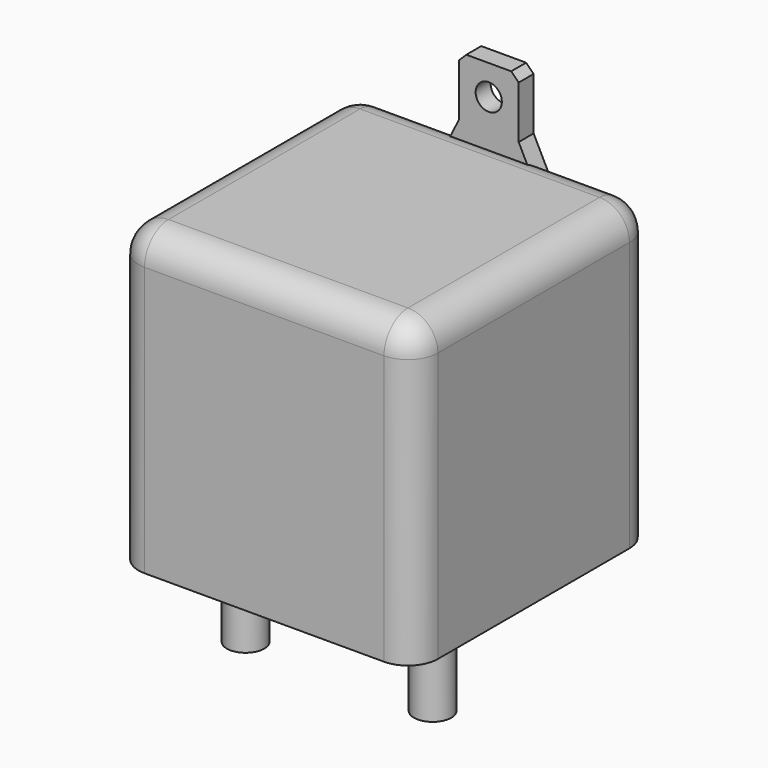
from build123d import *

# Parameters (mm, degrees)
F0_W         = 50.8
F0_H         = 50.8
F1_DEPTH     = 50.8
F2_R         = 2.2225
F3_DEPTH     = 3.175
F5_R         = 5.08
F6_T1_DEPTH  = 40.64
F6_T3_DEPTH  = 58.42
F6_T6_ANGLE  = 90
F6_T10_DEPTH = 26.67
F6_T16_DEPTH = 26.67
F6_T22_DEPTH = 26.67
F6_T27_ANGLE = 90
F6_T31_DEPTH = 26.67
F6_T38_DEPTH = 26.67
F6_T44_DEPTH = 26.67
F6_T48_ANGLE = 90
F6_T50_ANGLE = 90
F7_R         = 3.175
F8_DEPTH     = 15.24
F7_W         = 1.27
F7_H         = 6.35
F9_DEPTH     = 8.255


# Not quite as in the source:
# - a fillet or chamfer that OpenCascade refuses, or shapes differently, is made with other operations: its cross-section is extruded or revolved along the edge and cut away or added
# - a feature of the source that left no trace in its solid (it failed there, or was rolled back) is left out


with BuildPart() as f1:
    # F0 (on Top) → F1 (new body)
    with BuildSketch(Plane.XY):
        with Locations((-4.6946440548, -2.4632510453)):
            Rectangle(F0_W, F0_H)
    extrude(amount=F1_DEPTH)

    # F2 (on face) → F3 (join)
    with BuildSketch(Plane(origin=(0, 22.9367489547, 0), x_dir=(-1, 0, 0), z_dir=(0, 1, 0))):
        Polygon((-0.3853559452, 62.23), (-0.3853559452, 53.34), (9.7746440548, 53.34), (9.7746440548, 62.23), (8.5046440548, 63.5), (0.8846440548, 63.5), align=None)
        with Locations((4.6946440548, 58.42)):
            Circle(F2_R, mode=Mode.SUBTRACT)
        Polygon((-0.3853559452, 53.34), (-1.6553559452, 50.8), (11.0446440548, 50.8), (9.7746440548, 53.34), align=None)
    extrude(amount=-F3_DEPTH)

    # F5
    f5_edges = [f1.edges().sort_by_distance(p)[0] for p in [
        (-30.094644, -2.463251, 50.8),
        (20.705356, -2.463251, 50.8),
    ]]
    fillet(f5_edges, radius=F5_R)

    # F6: fillet of radius 5.08 on 11 edges, made by hand

    # F6_s2 → F6_t1 (cut)
    with BuildSketch(Plane.YZ.offset(-25.0146440548)):
        with BuildLine():
            ThreePointArc((-27.8632510453, 45.72), (-26.3753534938, 49.3121024484), (-22.7832510453, 50.8))
            Line((-22.7832510453, 50.8), (-27.8632510453, 50.8))
            Line((-27.8632510453, 50.8), (-27.8632510453, 45.72))
        make_face()
    extrude(amount=F6_T1_DEPTH, mode=Mode.SUBTRACT)

    # F6_s4 → F6_t3 (cut)
    with BuildSketch(Plane.XY.offset(-12.7)):
        with BuildLine():
            ThreePointArc((-30.0946440548, 17.8567489547), (-28.6067465032, 21.4488514031), (-25.0146440548, 22.9367489547))
            Line((-25.0146440548, 22.9367489547), (-30.0946440548, 22.9367489547))
            Line((-30.0946440548, 22.9367489547), (-30.0946440548, 17.8567489547))
        make_face()
        with BuildLine():
            ThreePointArc((-30.0946440548, -22.7832510453), (-28.6067465032, -26.3753534938), (-25.0146440548, -27.8632510453))
            Line((-25.0146440548, -27.8632510453), (-30.0946440548, -27.8632510453))
            Line((-30.0946440548, -27.8632510453), (-30.0946440548, -22.7832510453))
        make_face()
        with BuildLine():
            ThreePointArc((15.6253559452, 22.9367489547), (19.2174583937, 21.4488514031), (20.7053559452, 17.8567489547))
            Line((20.7053559452, 17.8567489547), (20.7053559452, 22.9367489547))
            Line((20.7053559452, 22.9367489547), (15.6253559452, 22.9367489547))
        make_face()
        with BuildLine():
            ThreePointArc((15.6253559452, -27.8632510453), (19.2174583937, -26.3753534938), (20.7053559452, -22.7832510453))
            Line((20.7053559452, -22.7832510453), (20.7053559452, -27.8632510453))
            Line((20.7053559452, -27.8632510453), (15.6253559452, -27.8632510453))
        make_face()
    extrude(amount=F6_T3_DEPTH, mode=Mode.SUBTRACT)

    # F6_s5 → F6_t6 (revolve, cut)
    with BuildSketch(Plane.YZ.offset(15.6253559452)):
        with BuildLine():
            ThreePointArc((22.9367489547, 45.72), (21.4488514031, 49.3121024484), (17.8567489547, 50.8))
            Line((17.8567489547, 50.8), (22.9367489547, 50.8))
            Line((22.9367489547, 50.8), (22.9367489547, 45.72))
        make_face()
    revolve(axis=Axis((15.6253559452, 22.9367489547, 45.72), (0, 1, 0)), revolution_arc=F6_T6_ANGLE, mode=Mode.SUBTRACT)


with BuildPart() as f6_tool8:
    # F6_s9 → F6_t10 (new body)
    with BuildSketch(Plane.YZ.offset(15.6253559452)):
        with BuildLine():
            ThreePointArc((22.9367489547, 45.72), (21.4488514031, 49.3121024484), (17.8567489547, 50.8))
            Line((17.8567489547, 50.8), (22.9367489547, 50.8))
            Line((22.9367489547, 50.8), (22.9367489547, 45.72))
        make_face()
    extrude(amount=-F6_T10_DEPTH)

    split(bisect_by=Plane.XZ.offset(-19.7617489547), keep=Keep.BOTTOM)

    split(bisect_by=Plane(origin=(21.6442847562, 0, 10.8221423781), x_dir=(0, 1, 0), z_dir=(0.894427191, 0, 0.4472135955)), keep=Keep.TOP)


with BuildPart() as f1_1:
    add(f1.part)

    # F6_t7: cut F6_tool8
    add(f6_tool8.part, mode=Mode.SUBTRACT)


with BuildPart() as f6_tool14:
    # F6_s15 → F6_t16 (new body)
    with BuildSketch(Plane.YZ.offset(15.6253559452)):
        with BuildLine():
            ThreePointArc((22.9367489547, 45.72), (21.4488514031, 49.3121024484), (17.8567489547, 50.8))
            Line((17.8567489547, 50.8), (22.9367489547, 50.8))
            Line((22.9367489547, 50.8), (22.9367489547, 45.72))
        make_face()
    extrude(amount=-F6_T16_DEPTH)

    split(bisect_by=Plane.XZ.offset(-19.7617489547), keep=Keep.TOP)

    split(bisect_by=Plane(origin=(21.6442847562, 0, 10.8221423781), x_dir=(0, 1, 0), z_dir=(0.894427191, 0, 0.4472135955)), keep=Keep.TOP)


with BuildPart() as f1_2:
    add(f1_1.part)

    # F6_t13: cut F6_tool14
    add(f6_tool14.part, mode=Mode.SUBTRACT)


with BuildPart() as f6_tool20:
    # F6_s21 → F6_t22 (new body)
    with BuildSketch(Plane.YZ.offset(15.6253559452)):
        with BuildLine():
            ThreePointArc((22.9367489547, 45.72), (21.4488514031, 49.3121024484), (17.8567489547, 50.8))
            Line((17.8567489547, 50.8), (22.9367489547, 50.8))
            Line((22.9367489547, 50.8), (22.9367489547, 45.72))
        make_face()
    extrude(amount=-F6_T22_DEPTH)

    split(bisect_by=Plane(origin=(-29.1557152438, 0, 14.5778576219), x_dir=(0, 1, 0), z_dir=(0.894427191, 0, -0.4472135955)), keep=Keep.TOP)

    split(bisect_by=Plane.XZ.offset(-19.7617489547), keep=Keep.TOP)

    split(bisect_by=Plane(origin=(21.6442847562, 0, 10.8221423781), x_dir=(0, 1, 0), z_dir=(-0.894427191, 0, -0.4472135955)), keep=Keep.TOP)


with BuildPart() as f1_3:
    add(f1_2.part)

    # F6_t19: cut F6_tool20
    add(f6_tool20.part, mode=Mode.SUBTRACT)

    # F6_s26 → F6_t27 (revolve, cut)
    with BuildSketch(Plane.XY.offset(45.72)):
        with BuildLine():
            ThreePointArc((-25.0146440548, 22.9367489547), (-28.6067465032, 21.4488514031), (-30.0946440548, 17.8567489547))
            Line((-30.0946440548, 17.8567489547), (-30.0946440548, 22.9367489547))
            Line((-30.0946440548, 22.9367489547), (-25.0146440548, 22.9367489547))
        make_face()
    revolve(axis=Axis((-25.0146440548, 22.9367489547, 45.72), (0, 1, 0)), revolution_arc=F6_T27_ANGLE, mode=Mode.SUBTRACT)


with BuildPart() as f6_tool29:
    # F6_s30 → F6_t31 (new body)
    with BuildSketch(Plane.YZ.offset(1.6553559452)):
        with BuildLine():
            ThreePointArc((22.9367489547, 45.72), (21.4488514031, 49.3121024484), (17.8567489547, 50.8))
            Line((17.8567489547, 50.8), (22.9367489547, 50.8))
            Line((22.9367489547, 50.8), (22.9367489547, 45.72))
        make_face()
    extrude(amount=-F6_T31_DEPTH)

    split(bisect_by=Plane(origin=(-29.1557152438, 0, 14.5778576219), x_dir=(0, 1, 0), z_dir=(0.894427191, 0, -0.4472135955)), keep=Keep.TOP)

    split(bisect_by=Plane.XZ.offset(-19.7617489547), keep=Keep.TOP)

    split(bisect_by=Plane(origin=(21.6442847562, 0, 10.8221423781), x_dir=(0, 1, 0), z_dir=(-0.894427191, 0, -0.4472135955)), keep=Keep.TOP)


with BuildPart() as f1_4:
    add(f1_3.part)

    # F6_t28: cut F6_tool29
    add(f6_tool29.part, mode=Mode.SUBTRACT)


with BuildPart() as f6_tool36:
    # F6_s37 → F6_t38 (new body)
    with BuildSketch(Plane.YZ.offset(1.6553559452)):
        with BuildLine():
            ThreePointArc((22.9367489547, 45.72), (21.4488514031, 49.3121024484), (17.8567489547, 50.8))
            Line((17.8567489547, 50.8), (22.9367489547, 50.8))
            Line((22.9367489547, 50.8), (22.9367489547, 45.72))
        make_face()
    extrude(amount=-F6_T38_DEPTH)

    split(bisect_by=Plane(origin=(-29.1557152438, 0, 14.5778576219), x_dir=(0, 1, 0), z_dir=(-0.894427191, 0, 0.4472135955)), keep=Keep.TOP)

    split(bisect_by=Plane.XZ.offset(-19.7617489547), keep=Keep.BOTTOM)


with BuildPart() as f1_5:
    add(f1_4.part)

    # F6_t35: cut F6_tool36
    add(f6_tool36.part, mode=Mode.SUBTRACT)


with BuildPart() as f6_tool42:
    # F6_s43 → F6_t44 (new body)
    with BuildSketch(Plane.YZ.offset(1.6553559452)):
        with BuildLine():
            ThreePointArc((22.9367489547, 45.72), (21.4488514031, 49.3121024484), (17.8567489547, 50.8))
            Line((17.8567489547, 50.8), (22.9367489547, 50.8))
            Line((22.9367489547, 50.8), (22.9367489547, 45.72))
        make_face()
    extrude(amount=-F6_T44_DEPTH)

    split(bisect_by=Plane(origin=(-29.1557152438, 0, 14.5778576219), x_dir=(0, 1, 0), z_dir=(-0.894427191, 0, 0.4472135955)), keep=Keep.TOP)

    split(bisect_by=Plane.XZ.offset(-19.7617489547), keep=Keep.TOP)


with BuildPart() as f1_6:
    add(f1_5.part)

    # F6_t41: cut F6_tool42
    add(f6_tool42.part, mode=Mode.SUBTRACT)

    # F6_s47 → F6_t48 (revolve, cut)
    with BuildSketch(Plane.XY.offset(45.72)):
        with BuildLine():
            ThreePointArc((-30.0946440548, -22.7832510453), (-28.6067465032, -26.3753534938), (-25.0146440548, -27.8632510453))
            Line((-25.0146440548, -27.8632510453), (-30.0946440548, -27.8632510453))
            Line((-30.0946440548, -27.8632510453), (-30.0946440548, -22.7832510453))
        make_face()
    revolve(axis=Axis((-25.0146440548, -27.8632510453, 45.72), (0, 1, 0)), revolution_arc=F6_T48_ANGLE, mode=Mode.SUBTRACT)

    # F6_s49 → F6_t50 (revolve, cut)
    with BuildSketch(Plane.YZ.offset(15.6253559452)):
        with BuildLine():
            ThreePointArc((-27.8632510453, 45.72), (-26.3753534938, 49.3121024484), (-22.7832510453, 50.8))
            Line((-22.7832510453, 50.8), (-27.8632510453, 50.8))
            Line((-27.8632510453, 50.8), (-27.8632510453, 45.72))
        make_face()
    revolve(axis=Axis((15.6253559452, -27.8632510453, 45.72), (0, 1, 0)), revolution_arc=F6_T50_ANGLE, mode=Mode.SUBTRACT)

    # F7 (on face) → F8 (join)
    with BuildSketch(Plane(origin=(0, 0, 0), x_dir=(1, 0, 0), z_dir=(0, 0, -1))):
        with Locations((-20.5696440548, 11.9882510453)):
            Circle(F7_R)
        with Locations((11.1803559452, 11.9882510453)):
            Circle(F7_R)
    extrude(amount=F8_DEPTH)

    # F7 (on face) → F9 (join)
    with BuildSketch(Plane(origin=(0, 0, 0), x_dir=(1, 0, 0), z_dir=(0, 0, -1))):
        with Locations((-7.8696440548, -7.0617489547)):
            Rectangle(F7_W, F7_H)
        with Locations((-1.5196440548, -7.0617489547)):
            Rectangle(F7_W, F7_H)
    extrude(amount=F9_DEPTH)


solid = f1_6.part
